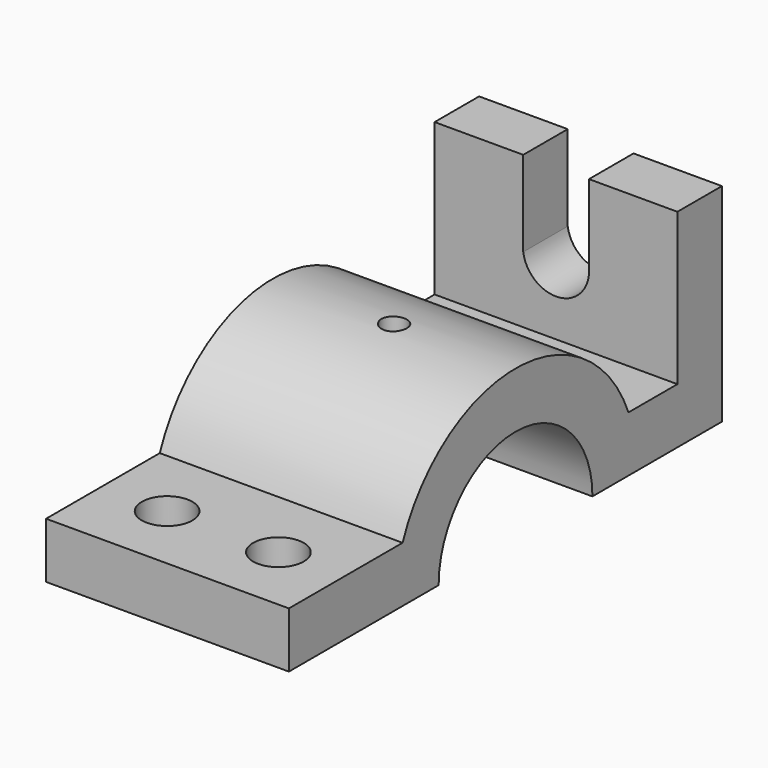
from build123d import *

# Parameters (mm, degrees)
F0_W     = 11
F0_H     = 30
F1_DEPTH = 24
F3_DEPTH = 11
F4_R     = 5
F4_R_2   = 2.5
F5_DEPTH = 41.001


with BuildPart() as f1:
    # F0 (on Right) → F1 (new body, symmetric)
    with BuildSketch(Plane.YZ):
        with BuildLine():
            Line((-56, 0), (-30, 0))
            ThreePointArc((-30, 0), (-29.4730143031, 5.5983415304), (-27.9105714739, 11))
            Line((-27.9105714739, 11), (-56, 11))
            Line((-56, 11), (-56, 0))
        make_face()
        with BuildLine():
            ThreePointArc((-27.9105714739, 11), (-29.4730143031, 5.5983415304), (-30, 0))
            Line((-30, 0), (-19, 0))
            ThreePointArc((-19, 0), (-18.1017503893, 5.7729223833), (-15.4919333848, 11))
            Line((-15.4919333848, 11), (-27.9105714739, 11))
        make_face()
        with BuildLine():
            Line((15.4919333848, 11), (27.9105714739, 11))
            ThreePointArc((27.9105714739, 11), (0, 30), (-27.9105714739, 11))
            Line((-27.9105714739, 11), (-15.4919333848, 11))
            ThreePointArc((-15.4919333848, 11), (0, 19), (15.4919333848, 11))
        make_face()
        with BuildLine():
            Line((19, 0), (30, 0))
            ThreePointArc((30, 0), (29.4730143031, 5.5983415304), (27.9105714739, 11))
            Line((27.9105714739, 11), (15.4919333848, 11))
            ThreePointArc((15.4919333848, 11), (18.1017503893, 5.7729223833), (19, 0))
        make_face()
        with BuildLine():
            ThreePointArc((27.9105714739, 11), (29.4730143031, 5.5983415304), (30, 0))
            Line((30, 0), (51, 0))
            Line((51, 0), (51, 11))
            Line((51, 11), (40, 11))
            Line((40, 11), (27.9105714739, 11))
        make_face()
        with Locations((45.5, 26)):
            Rectangle(F0_W, F0_H)
    extrude(amount=F1_DEPTH, both=True)

    # F2 (on face) → F3 (cut, through all)
    with BuildSketch(Plane(origin=(0, 51, 0), x_dir=(-1, 0, 0), z_dir=(0, 1, 0))):
        with BuildLine():
            Line((-6.5220605694, 25.4945768912), (-6.5220605694, 24.5054231088))
            ThreePointArc((-6.5220605694, 24.5054231088), (-0.2061620785, 18.4624639527), (6.4779394306, 24.0954663604))
            Line((6.4779394306, 24.0954663604), (6.4779394306, 25.9045336396))
            ThreePointArc((6.4779394306, 25.9045336396), (-0.2061620785, 31.5375360473), (-6.5220605694, 25.4945768912))
        make_face()
        with BuildLine():
            Line((-6.5220605694, 41), (-6.5220605694, 25.4945768912))
            ThreePointArc((-6.5220605694, 25.4945768912), (-0.2061620785, 31.5375360473), (6.4779394306, 25.9045336396))
            Line((6.4779394306, 25.9045336396), (6.4779394306, 41))
            Line((6.4779394306, 41), (-6.5220605694, 41))
        make_face()
    extrude(amount=-F3_DEPTH, mode=Mode.SUBTRACT)

    # F4 (on Top) → F5 (cut, through all)
    with BuildSketch(Plane.XY):
        with Locations((11, -42.3406362534)):
            Circle(F4_R)
        with Locations((-11, -42.3406362534)):
            Circle(F4_R)
        Circle(F4_R_2)
    extrude(amount=F5_DEPTH, mode=Mode.SUBTRACT)


solid = f1.part
